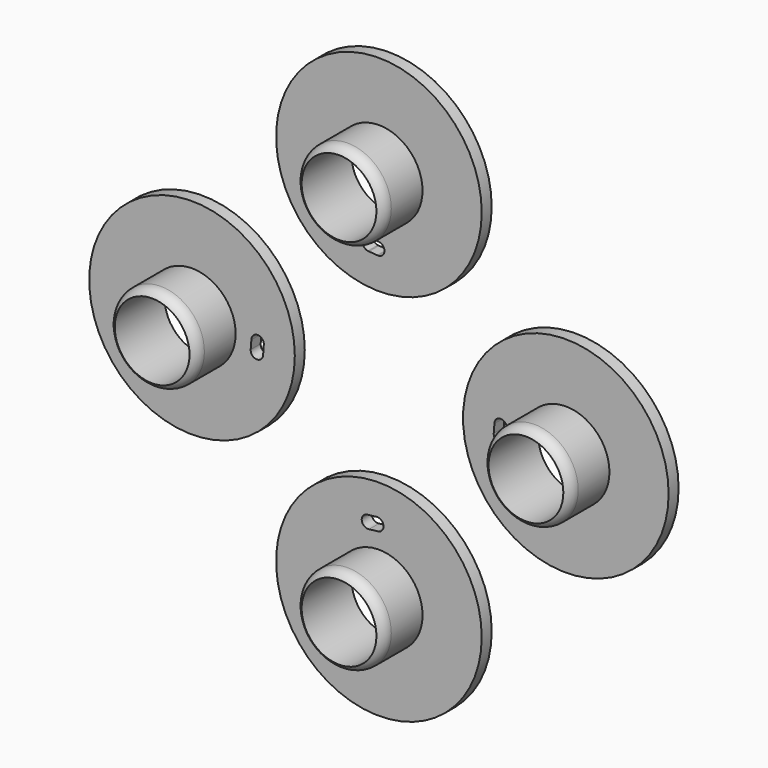
from build123d import *

# Parameters (mm, degrees)
F0_R     = 7
F0_R_2   = 6
F1_DEPTH = 10
F0_R_3   = 16.5
F0_R_4   = 12.5
F2_DEPTH = 2


# Not quite as in the source:
# - a fillet or chamfer that OpenCascade refuses, or shapes differently, is made with other operations: its cross-section is extruded or revolved along the edge and cut away or added


with BuildPart() as f1:
    # F0 (on Front) → F1 (new body)
    with BuildSketch(Plane.XZ):
        with Locations((-30, 0)):
            Circle(F0_R)
        with Locations((-30, 0)):
            Circle(F0_R_2, mode=Mode.SUBTRACT)
    extrude(amount=F1_DEPTH)

    # F3: fillet of radius 2 on 1 edges, made by hand

    # F3_s1 → F3_t2 (revolve, cut)
    with BuildSketch(Plane.XY):
        with BuildLine():
            ThreePointArc((-23, -8.2679491924), (-23.2679491924, -9.2679491924), (-24, -10))
            Line((-24, -10), (-23, -10))
            Line((-23, -10), (-23, -8.2679491924))
        make_face()
    revolve(axis=Axis((-30, -10, 0), (0, -1, 0)), mode=Mode.SUBTRACT)


with BuildPart() as f1b:
    # F0 (on Front) → F1, piece 2 (new body)
    with BuildSketch(Plane.XZ):
        with Locations((0, 30)):
            Circle(F0_R)
        with Locations((0, 30)):
            Circle(F0_R_2, mode=Mode.SUBTRACT)
    extrude(amount=F1_DEPTH)

    # F3#2: fillet of radius 2 on 1 edges, made by hand

    # F3_2_s1 → F3_2_t2 (revolve, cut)
    with BuildSketch(Plane.XY.offset(30)):
        with BuildLine():
            ThreePointArc((7, -8.2679491924), (6.7320508076, -9.2679491924), (6, -10))
            Line((6, -10), (7, -10))
            Line((7, -10), (7, -8.2679491924))
        make_face()
    revolve(axis=Axis((0, -10, 30), (0, -1, 0)), mode=Mode.SUBTRACT)


with BuildPart() as f1c:
    # F0 (on Front) → F1, piece 3 (new body)
    with BuildSketch(Plane.XZ):
        with Locations((30, 0)):
            Circle(F0_R)
        with Locations((30, 0)):
            Circle(F0_R_2, mode=Mode.SUBTRACT)
    extrude(amount=F1_DEPTH)

    # F3#3: fillet of radius 2 on 1 edges, made by hand

    # F3_3_s1 → F3_3_t2 (revolve, cut)
    with BuildSketch(Plane.XY):
        with BuildLine():
            ThreePointArc((37, -8.2679491924), (36.7320508076, -9.2679491924), (36, -10))
            Line((36, -10), (37, -10))
            Line((37, -10), (37, -8.2679491924))
        make_face()
    revolve(axis=Axis((30, -10, 0), (0, -1, 0)), mode=Mode.SUBTRACT)


with BuildPart() as f1d:
    # F0 (on Front) → F1, piece 4 (new body)
    with BuildSketch(Plane.XZ):
        with Locations((0, -30)):
            Circle(F0_R)
        with Locations((0, -30)):
            Circle(F0_R_2, mode=Mode.SUBTRACT)
    extrude(amount=F1_DEPTH)

    # F3#4: fillet of radius 2 on 1 edges, made by hand

    # F3_4_s1 → F3_4_t2 (revolve, cut)
    with BuildSketch(Plane.XY.offset(-30)):
        with BuildLine():
            ThreePointArc((7, -8.2679491924), (6.7320508076, -9.2679491924), (6, -10))
            Line((6, -10), (7, -10))
            Line((7, -10), (7, -8.2679491924))
        make_face()
    revolve(axis=Axis((0, -10, -30), (0, -1, 0)), mode=Mode.SUBTRACT)


with BuildPart() as f2:
    # F0 (on Front) → F2 (new body)
    with BuildSketch(Plane.XZ):
        with Locations((-30, 0)):
            Circle(F0_R_3)
        with Locations((-30, 0)):
            Circle(F0_R_4, mode=Mode.SUBTRACT)
        with Locations((-30, 0)):
            Circle(F0_R_4)
        with BuildLine():
            ThreePointArc((-20.4715704369, 0), (-19.4715704369, 1), (-18.4715704369, 0))
            ThreePointArc((-18.4715704369, 0), (-18.4744598192, -0.0759632549), (-18.4831112691, -0.151487536))
            Line((-18.4831112691, -0.151487536), (-18.5848039346, -1.4863281334))
            ThreePointArc((-18.5848039346, -1.4863281334), (-18.5847338366, -1.493163907), (-18.5847104703, -1.5))
            ThreePointArc((-18.5847104703, -1.5), (-18.5881424433, -1.5827778208), (-18.5984148055, -1.6649874592))
            ThreePointArc((-18.5984148055, -1.6649874592), (-19.7059181598, -2.4926271687), (-20.5817268135, -1.4228092539))
            Line((-20.5817268135, -1.4228092539), (-20.4715704369, 0))
        make_face(mode=Mode.SUBTRACT)
        with Locations((-30, 0)):
            Circle(F0_R, mode=Mode.SUBTRACT)
    extrude(amount=F2_DEPTH)


with BuildPart() as f2b:
    # F0 (on Front) → F2, piece 2 (new body)
    with BuildSketch(Plane.XZ):
        with Locations((0, 30)):
            Circle(F0_R_3)
        with Locations((0, 30)):
            Circle(F0_R_4, mode=Mode.SUBTRACT)
        with Locations((0, 30)):
            Circle(F0_R_4)
        with BuildLine():
            ThreePointArc((-0.1136225039, 20.5006795018), (0.5934842773, 20.207786283), (0.8863774961, 19.5006795018))
            ThreePointArc((0.8863774961, 19.5006795018), (0.5934842773, 18.7935727207), (-0.1136225039, 18.5006795018))
            ThreePointArc((-0.1136225039, 18.5006795018), (-0.1895857587, 18.5035688842), (-0.2651100399, 18.512220334))
            Line((-0.2651100399, 18.512220334), (-1.5999506373, 18.6139129995))
            ThreePointArc((-1.5999506373, 18.6139129995), (-1.6895857587, 18.6167089175), (-1.7786099631, 18.6275238705))
            ThreePointArc((-1.7786099631, 18.6275238705), (-2.6062496725, 19.7350272248), (-1.5364317578, 20.6108358785))
            Line((-1.5364317578, 20.6108358785), (-0.1136225039, 20.5006795018))
        make_face(mode=Mode.SUBTRACT)
        with Locations((0, 30)):
            Circle(F0_R, mode=Mode.SUBTRACT)
    extrude(amount=F2_DEPTH)


with BuildPart() as f2c:
    # F0 (on Front) → F2, piece 3 (new body)
    with BuildSketch(Plane.XZ):
        with Locations((30, 0)):
            Circle(F0_R_3)
        with Locations((30, 0)):
            Circle(F0_R_4, mode=Mode.SUBTRACT)
        with Locations((30, 0)):
            Circle(F0_R_4)
        with BuildLine():
            ThreePointArc((18.5373204914, 0.8412470011), (19.5373204914, 1.8412470011), (20.5373204914, 0.8412470011))
            ThreePointArc((20.5373204914, 0.8412470011), (20.5344311091, 0.7652837462), (20.5257796592, 0.6897594651))
            Line((20.5257796592, 0.6897594651), (20.4240869937, -0.6450811323))
            ThreePointArc((20.4240869937, -0.6450811323), (20.4241570916, -0.6519169059), (20.424180458, -0.6587529989))
            ThreePointArc((20.424180458, -0.6587529989), (20.420748485, -0.7415308198), (20.4104761228, -0.8237404581))
            ThreePointArc((20.4104761228, -0.8237404581), (19.3029727684, -1.6513801676), (18.4271641147, -0.5815622529))
            Line((18.4271641147, -0.5815622529), (18.5373204914, 0.8412470011))
        make_face(mode=Mode.SUBTRACT)
        with Locations((30, 0)):
            Circle(F0_R, mode=Mode.SUBTRACT)
    extrude(amount=F2_DEPTH)


with BuildPart() as f2d:
    # F0 (on Front) → F2, piece 4 (new body)
    with BuildSketch(Plane.XZ):
        with Locations((0, -30)):
            Circle(F0_R_3)
        with Locations((0, -30)):
            Circle(F0_R_4, mode=Mode.SUBTRACT)
        with Locations((0, -30)):
            Circle(F0_R_4)
        with BuildLine():
            ThreePointArc((-1.5777100629, -20.6319249065), (-2.7433591479, -19.8311364135), (-1.9425706549, -18.6654873284))
            ThreePointArc((-1.9425706549, -18.6654873284), (-1.8729385877, -18.6550882032), (-1.8027474061, -18.64961421))
            Line((-1.8027474061, -18.64961421), (-0.4411743003, -18.4950446993))
            ThreePointArc((-0.4411743003, -18.4950446993), (-0.3729385877, -18.4849036338), (-0.3041660736, -18.4794911499))
            ThreePointArc((-0.3041660736, -18.4794911499), (0.4312257834, -18.7560169755), (0.7398596411, -19.4785215481))
            ThreePointArc((0.7398596411, -19.4785215481), (0.4851842917, -20.1452232545), (-0.1491226894, -20.4723399807))
            Line((-0.1491226894, -20.4723399807), (-1.5777100629, -20.6319249065))
        make_face(mode=Mode.SUBTRACT)
        with Locations((0, -30)):
            Circle(F0_R, mode=Mode.SUBTRACT)
    extrude(amount=F2_DEPTH)


solid = Compound([f1.part, f1b.part, f1c.part, f1d.part, f2.part, f2b.part, f2c.part, f2d.part])
